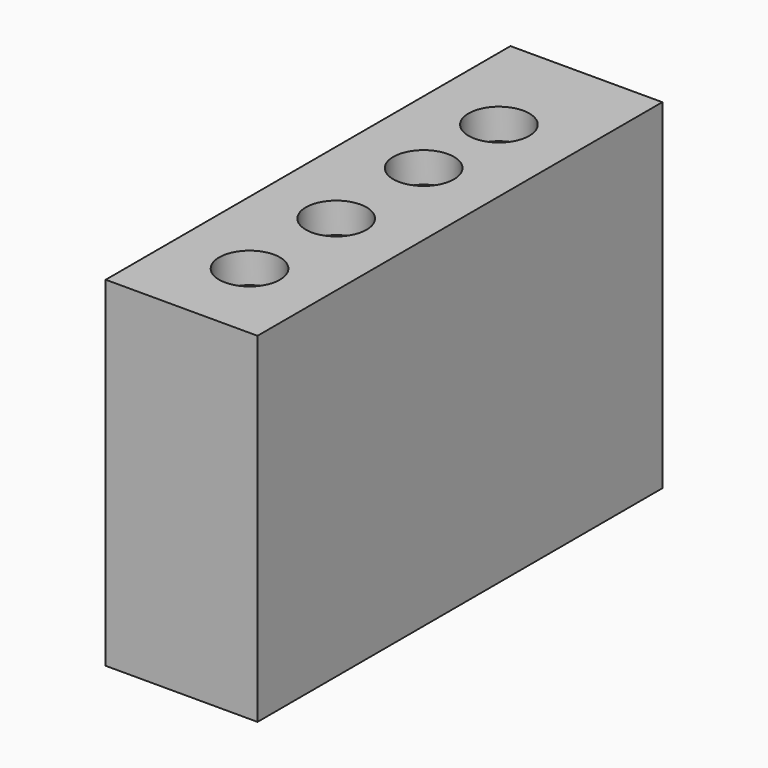
from build123d import *

# Parameters (mm, degrees)
F0_W           = 83.3091139793
F0_H           = 55.9713058174
F1_DEPTH       = 25
F3_D           = 5
F3_DEPTH       = 20
F3_CBORE_D     = 10
F3_CBORE_DEPTH = 5
F3_TIP         = 1.5021515476


with BuildPart() as f1:
    # F0 (on Right) → F1 (new body)
    with BuildSketch(Plane.YZ):
        Rectangle(F0_W, F0_H)
    extrude(amount=F1_DEPTH)

    # F3
    with Locations(Plane.XY.offset(27.9856529087)):
        with Locations((12.5, -27.6769809425), (12.5, -9.8345736042), (12.5, 8.1630079076), (12.5, 23.6527305096)):
            CounterBoreHole(F3_D / 2, F3_CBORE_D / 2, F3_CBORE_DEPTH, depth=F3_DEPTH)
            with Locations((0, 0, -(F3_DEPTH + F3_TIP / 2))):  # 118° drill point
                Cone(0, F3_D / 2, F3_TIP, mode=Mode.SUBTRACT)


solid = f1.part
